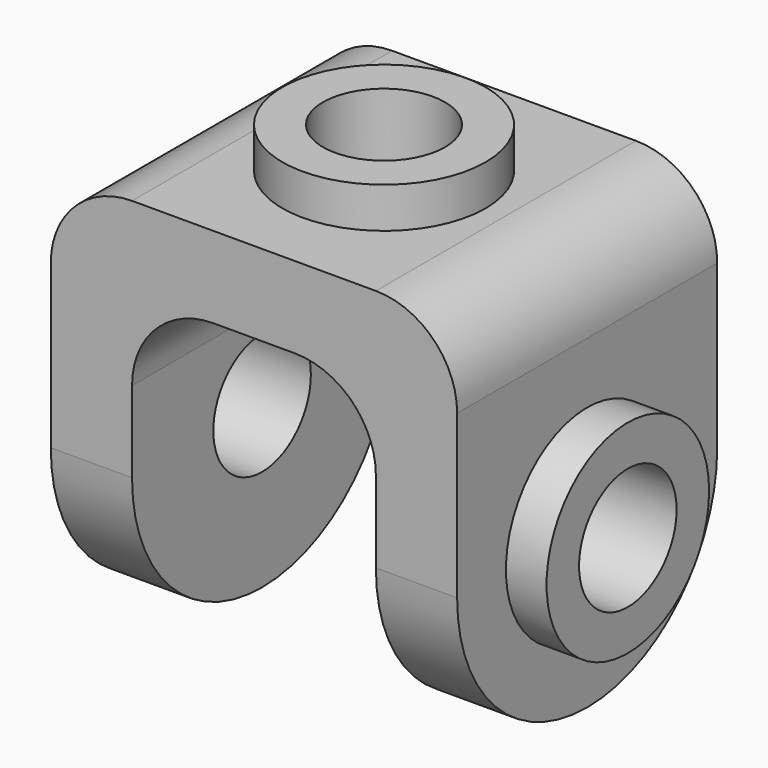
from build123d import *

# Parameters (mm, degrees)
F1_DEPTH  = 200
F2_R      = 199.99999
F3_R      = 125
F4_DEPTH  = 50
F5_R      = 125
F6_DEPTH  = 50
F7_R      = 75
F8_DEPTH  = 350
F9_R      = 75
F10_DEPTH = 312.5


# Not quite as in the source:
# - a fillet or chamfer is up to 0.001 mm smaller than in the source, because OpenCascade refuses the exact size
# - a pattern or mirror of a feature is missing from the dataset's text; its kind, count and spacing are read off the source's solid


with BuildPart() as f1:
    # F0 (on Front) → F1 (new body, symmetric)
    with BuildSketch(Plane.XZ):
        with BuildLine():
            ThreePointArc((250, 150), (220.7106781187, 220.7106781187), (150, 250))
            Line((150, 250), (-150, 250))
            ThreePointArc((-150, 250), (-220.7106781187, 220.7106781187), (-250, 150))
            Line((-250, 150), (-250, -250))
            Line((-250, -250), (-150, -250))
            Line((-150, -250), (-150, 50))
            ThreePointArc((-150, 50), (-120.7106781187, 120.7106781187), (-50, 150))
            Line((-50, 150), (50, 150))
            ThreePointArc((50, 150), (120.7106781187, 120.7106781187), (150, 50))
            Line((150, 50), (150, -250))
            Line((150, -250), (250, -250))
            Line((250, -250), (250, 150))
        make_face()
    extrude(amount=F1_DEPTH, both=True)

    # F2 (radius 200 in the source; OpenCascade refuses exactly that, so slightly less here)
    f2_edges = [f1.edges().sort_by_distance(p)[0] for p in [
        (-200, -200, -250),
        (-200, 200, -250),
        (200, -200, -250),
        (200, 200, -250),
    ]]
    fillet(f2_edges, radius=F2_R)

    # F3 (on face) → F4 (join)
    with BuildSketch(Plane.YZ.offset(250)):
        with Locations((0, -50)):
            Circle(F3_R)
    f4 = extrude(amount=F4_DEPTH)

    # F4_copies: F4 across plane
    add(f4.mirror(Plane(origin=(0, 0, 0), x_dir=(0, 0, -1), z_dir=(-1, 0, 0))))

    # F5 (on face) → F6 (join)
    with BuildSketch(Plane.XY.offset(250)):
        Circle(F5_R)
    extrude(amount=F6_DEPTH)

    # F7 (on Right) → F8 (cut, symmetric)
    with BuildSketch(Plane.YZ):
        with Locations((0, -50)):
            Circle(F7_R)
    extrude(amount=F8_DEPTH, both=True, mode=Mode.SUBTRACT)

    # F9 (on face) → F10 (cut)
    with BuildSketch(Plane.XY.offset(300)):
        Circle(F9_R)
    extrude(amount=-F10_DEPTH, mode=Mode.SUBTRACT)


solid = f1.part
